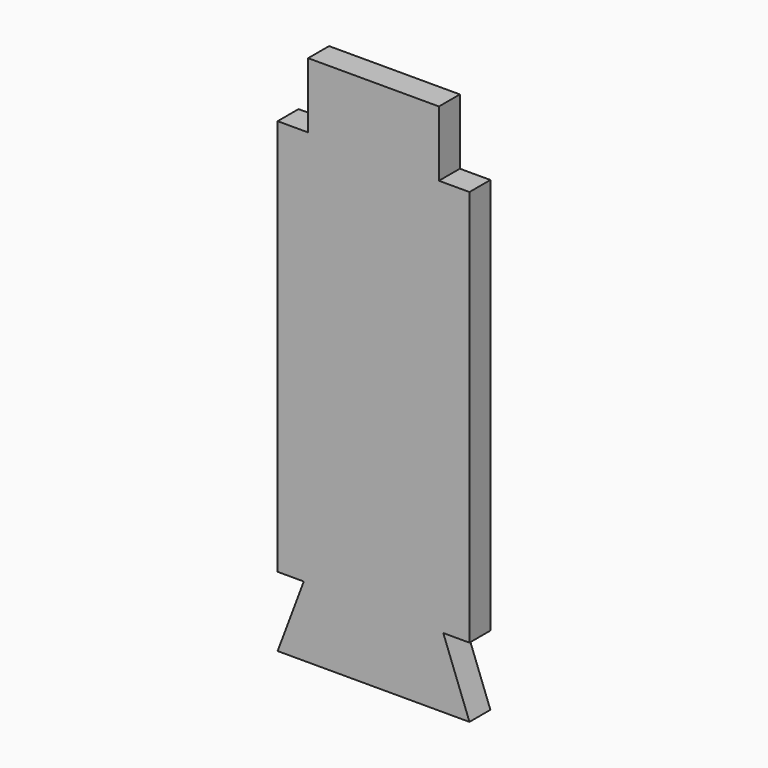
from build123d import *

# Parameters (mm, degrees)
F0_W     = 139.7
F0_H     = 387.35
F1_DEPTH = 19.05
F2_W     = 22.225
F2_H     = 47.625
F3_DEPTH = 19.051
F6_DEPTH = 19.051


# Not quite as in the source:
# - a length typed as a fraction of an inch, garbled in the dataset ("3 / 203.2 mm" for 3/8 in), is restored
# - a pattern or mirror of a feature is missing from the dataset's text; its kind, count and spacing are read off the source's solid


with BuildPart() as f1:
    # F0 (on Front) → F1 (new body)
    with BuildSketch(Plane.XZ):
        with Locations((69.85, 193.675)):
            Rectangle(F0_W, F0_H)
    extrude(amount=F1_DEPTH)

    # F2 (on face) → F3 (cut, through all)
    with BuildSketch(Plane.XZ.offset(19.05)):
        with Locations((11.1125, 363.5375)):
            Rectangle(F2_W, F2_H)
    f3 = extrude(amount=-F3_DEPTH, mode=Mode.SUBTRACT)

    # F3_copies: F3 across plane
    add(f3.mirror(Plane(origin=(69.85, 0, 0), x_dir=(0, 0, 1), z_dir=(1, 0, 0))), mode=Mode.SUBTRACT)

    # F5 (on face) → F6 (cut, through all)
    with BuildSketch(Plane.XZ.offset(19.05)):
        Polygon((0, 50.8), (0, 0), (19.05, 50.8), align=None)
    f6 = extrude(amount=-F6_DEPTH, mode=Mode.SUBTRACT)

    # F6_copies: F6 across plane
    add(f6.mirror(Plane(origin=(69.85, 0, 0), x_dir=(0, 0, 1), z_dir=(1, 0, 0))), mode=Mode.SUBTRACT)


solid = f1.part
